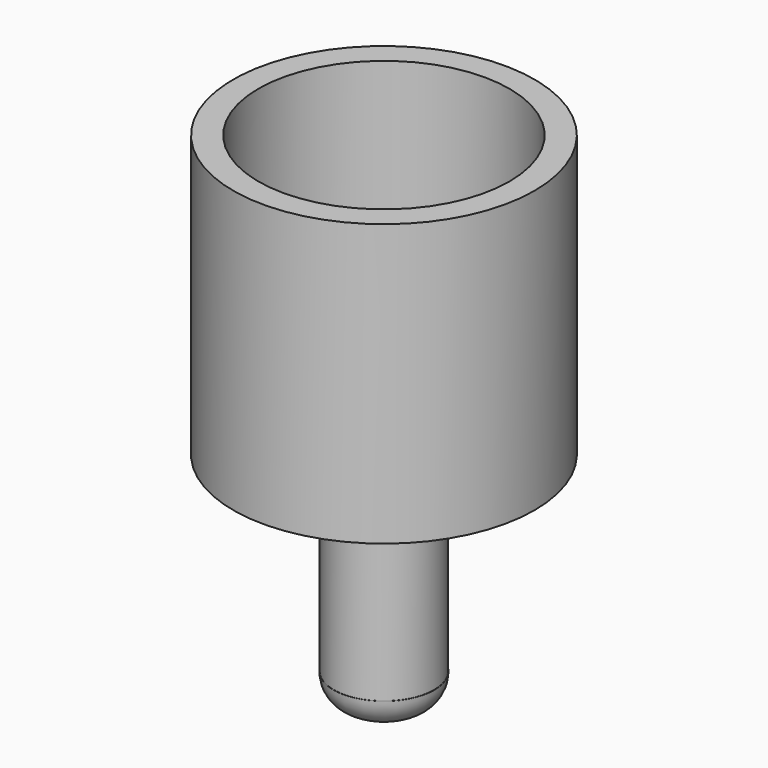
from build123d import *

# Parameters (mm, degrees)
F0_R     = 15
F0_R_2   = 12.5
F7_DEPTH = 25
F0_R_3   = 5
F1_DEPTH = 3
F0_R_4   = 3.25
F2_DEPTH = 22
F3_R     = 5.0189857481
F4_DEPTH = 3
F5_R     = 2.99999
F6_R     = 2


# Not quite as in the source:
# - a fillet or chamfer is up to 0.001 mm smaller than in the source, because OpenCascade refuses the exact size


with BuildPart() as f7:
    # F0 (on Top) → F7 (new body)
    with BuildSketch(Plane.XY):
        Circle(F0_R)
        Circle(F0_R_2, mode=Mode.SUBTRACT)
    extrude(amount=F7_DEPTH)

    # F0 (on Top) → F1 (join)
    with BuildSketch(Plane.XY):
        Circle(F0_R)
        Circle(F0_R_2, mode=Mode.SUBTRACT)
        Circle(F0_R_2)
        Circle(F0_R_3, mode=Mode.SUBTRACT)
    extrude(amount=-F1_DEPTH)

    # F0 (on Top) → F2 (join)
    with BuildSketch(Plane.XY):
        Circle(F0_R_3)
        Circle(F0_R_4, mode=Mode.SUBTRACT)
    extrude(amount=-F2_DEPTH)

    # F3 (on face) → F4 (join)
    with BuildSketch(Plane(origin=(0, 0, -22), x_dir=(1, 0, 0), z_dir=(0, 0, -1))):
        Circle(F3_R)
    extrude(amount=F4_DEPTH)

    # F5 (radius 3 in the source; OpenCascade refuses exactly that, so slightly less here)
    f5_edges = [f7.edges().sort_by_distance(p)[0] for p in [
        (-5.018986, 0, -25),
    ]]
    fillet(f5_edges, radius=F5_R)

    # F6
    f6_edges = [f7.edges().sort_by_distance(p)[0] for p in [
        (-3.25, 0, 0),
    ]]
    fillet(f6_edges, radius=F6_R)


solid = f7.part
